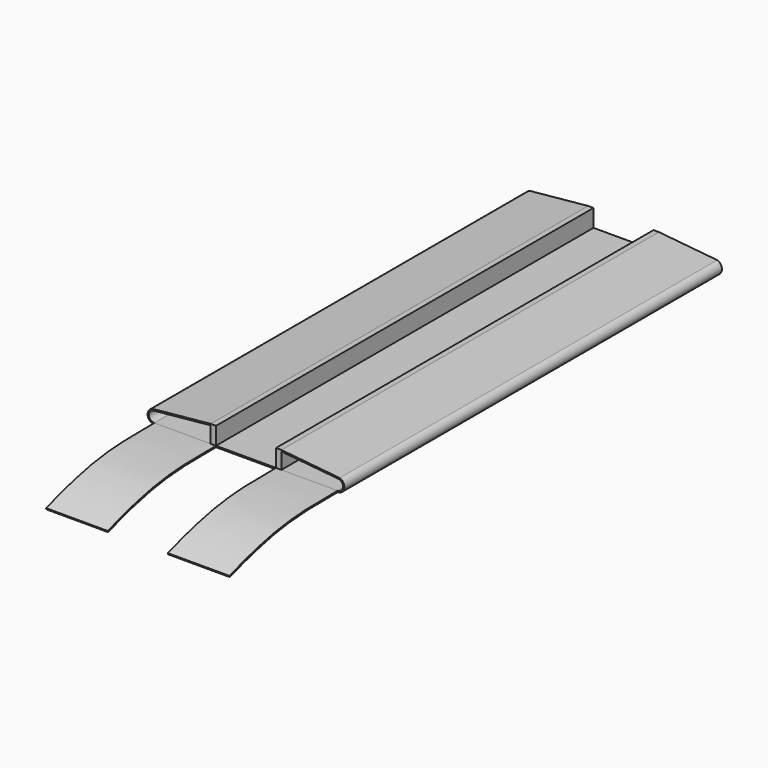
from build123d import *

# Parameters (mm, degrees)
F1_DEPTH = 350
F4_DEPTH = 45.75


with BuildPart() as f1:
    # F0 (on Front) → F1 (new body)
    with BuildSketch(Plane.XZ):
        with BuildLine():
            ThreePointArc((-69.4691266018, 9.7792956623), (-72.9445160689, 4.257193939), (-68, 0))
            Line((-68, 0), (0, 0))
            Line((0, 0), (68, 0))
            ThreePointArc((68, 0), (72.9445160689, 4.257193939), (69.4691266018, 9.7792956623))
            Line((69.4691266018, 9.7792956623), (26.3469652224, 13.9905305459))
            ThreePointArc((26.3469652224, 13.9905305459), (26.2498846097, 13.9976312337), (26.1525734896, 14))
            Line((26.1525734896, 14), (26.0150079844, 14))
            Line((26.0150079844, 14), (22.25, 14))
            Line((22.25, 14), (22.25, 1))
            Line((22.25, 1), (0, 1))
            Line((0, 1), (-22.25, 1))
            Line((-22.25, 1), (-22.25, 14))
            Line((-22.25, 14), (-26.0150079844, 14))
            Line((-26.0150079844, 14), (-26.1525734896, 14))
            ThreePointArc((-26.1525734896, 14), (-26.2498846097, 13.9976312337), (-26.3469652224, 13.9905305459))
            Line((-26.3469652224, 13.9905305459), (-69.4691266018, 9.7792956623))
        make_face()
        with BuildLine():
            Line((-26.25, 12.9720028672), (-26.25, 1))
            Line((-26.25, 1), (-68, 1))
            ThreePointArc((-68, 1), (-71.9482597731, 4.3587163152), (-69.265977288, 8.7943776178))
            Line((-69.265977288, 8.7943776178), (-26.25, 12.9952427487))
            Line((-26.25, 12.9952427487), (-26.25, 12.9720028672))
        make_face(mode=Mode.SUBTRACT)
        with BuildLine():
            Line((68, 1), (26.25, 1))
            Line((26.25, 1), (26.25, 12.9720028672))
            Line((26.25, 12.9720028672), (26.25, 12.9952427487))
            Line((26.25, 12.9952427487), (69.265977288, 8.7943776178))
            ThreePointArc((69.265977288, 8.7943776178), (71.9482597731, 4.3587163152), (68, 1))
        make_face(mode=Mode.SUBTRACT)
    extrude(amount=-F1_DEPTH)

    # F3 (on offset) → F4 (join)
    with BuildSketch(Plane.YZ.offset(-22.25)):
        with BuildLine():
            add(Edge.make_bspline(
                [(0, 0), (-36.9747690856, 0), (-56.282736361, 0), (-100.0474691391, -14.7872483358)],
                knots=[0, 0, 0, 0, 101.1343601081, 101.1343601081, 101.1343601081, 101.1343601081], degree=3))
            Line((0, 0), (0, 1))
            add(Edge.make_bspline(
                [(0, 1), (-9.2436922714, 1), (-25.5401100661, 1.0005275684), (-47.3845795682, -0.3908549289), (-70.5242758511, -4.5730687745), (-89.4052629561, -10.135915446), (-100.3675713535, -13.8398653233)],
                knots=[0, 0, 0, 0, 0.25, 0.5, 0.75, 1, 1, 1, 1], degree=3))
            Line((-100.3675713535, -13.8398653233), (-100.0474691391, -14.7872483358))
        make_face()
    extrude(amount=-F4_DEPTH)

    # F5: F1 across plane


with BuildPart() as f1_1:
    add(f1.part)
    add(f1.part.mirror(Plane.YZ))


solid = f1_1.part
